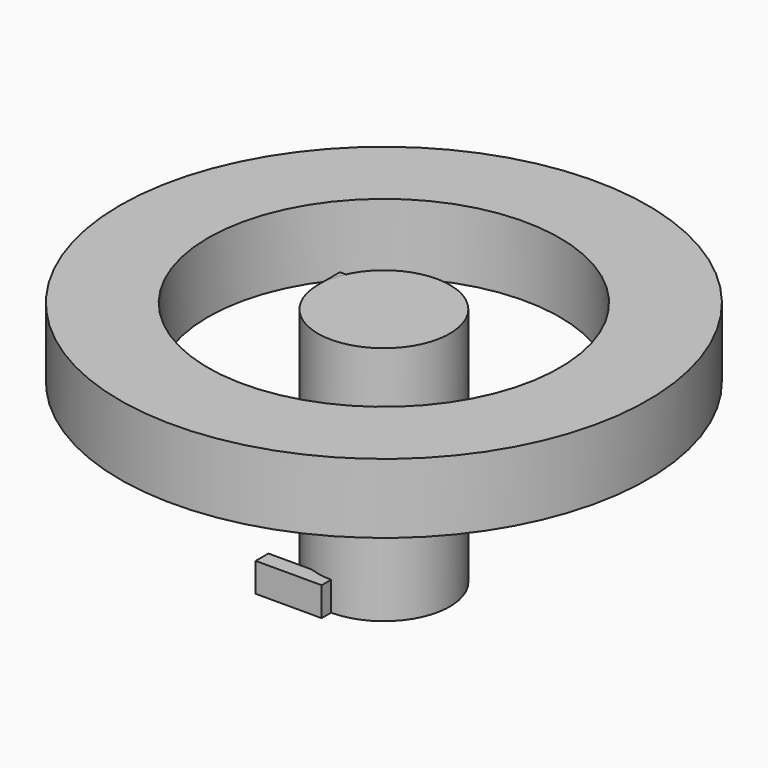
from build123d import *

# Parameters (mm, degrees)
F0_W      = 6.1436966062
F0_H      = 11.1728049815
F1_DEPTH  = 25.4
F0_W_2    = 10.5770677328
F0_H_2    = 92.550970614
F4_W      = 33.9257717133
F4_H      = 26.7906486988
F1_FACE_W = 25.4
F1_FACE_H = 92.550970614


# Not quite as in the source:
# - the program builds the solid bodies; features that only make, move or delete a surface that nothing else refers to are left out


with BuildPart() as f1:
    # F0 (on Right) → F1 (new body)
    with BuildSketch(Plane.YZ):
        with Locations((-26.9047878683, 44.6388516575)):
            Rectangle(F0_W, F0_H)
    extrude(amount=F1_DEPTH)


with BuildPart() as f1b:
    # F0 (on Right) → F1, piece 2 (new body)
    with BuildSketch(Plane.YZ):
        with Locations((5.2885338664, 85.3279344738)):
            Rectangle(F0_W_2, F0_H_2)
    extrude(amount=F1_DEPTH)


with BuildPart() as f5:
    # F4 (on Front) → F5 (revolve)
    with BuildSketch(Plane.XZ):
        with Locations((-59.2873692513, 120.3713193536)):
            Rectangle(F4_W, F4_H)
    revolve(axis=Axis((25.4, 0, 85.3279344738), (0, 0, 1)))


with BuildPart() as f5b:
    # F1_face (on face) → F5, piece 2 (revolve)
    with BuildSketch(Plane(origin=(12.7, 0, 85.3279344738), x_dir=(1, 0, 0), z_dir=(0, -1, 0))):
        Rectangle(F1_FACE_W, F1_FACE_H)
    revolve(axis=Axis((25.4, 0, 85.3279344738), (0, 0, 1)))


solid = Compound([f1.part, f1b.part, f5.part, f5b.part])
